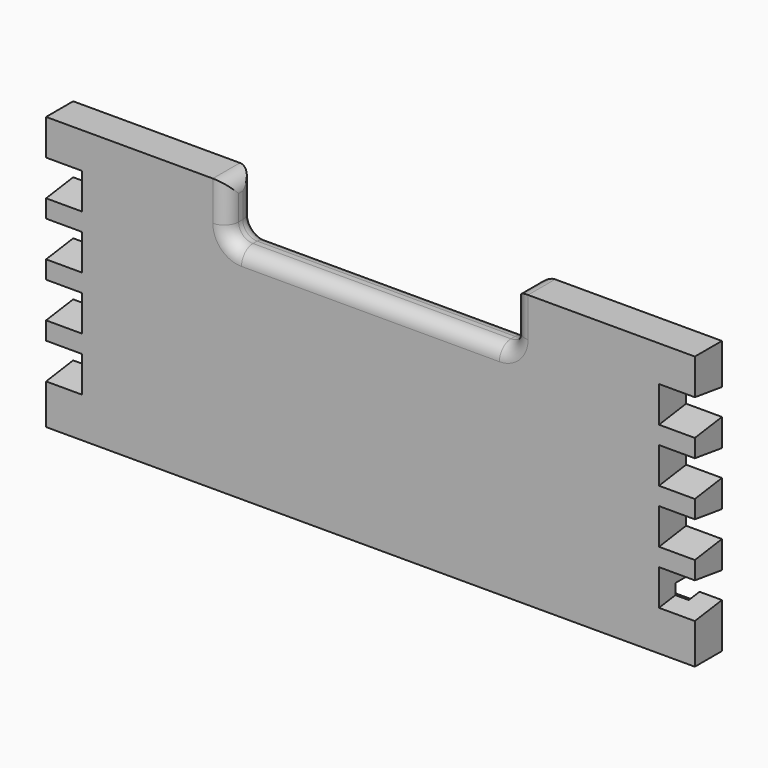
from build123d import *

# Parameters (mm, degrees)
F0_W     = 230
F0_H     = 96.8045385678
F1_DEPTH = 12
F2_W     = 101.6
F2_H     = 19.05
F3_DEPTH = 12
F4_R     = 5.08
F6_DEPTH = 12.7
F7_W     = 204.6
F7_H     = 6.35
F7_W_2   = 4.7625
F8_DEPTH = 4.7625


# Not quite as in the source:
# - a pattern or mirror of a feature is missing from the dataset's text; its kind, count and spacing are read off the source's solid


with BuildPart() as f1:
    # F0 (on Front) → F1 (new body)
    with BuildSketch(Plane.XZ):
        Rectangle(F0_W, F0_H)
    extrude(amount=-F1_DEPTH)

    # F2 (on face) → F3 (cut, through all)
    with BuildSketch(Plane.XZ):
        with Locations((0, 38.8772692839)):
            Rectangle(F2_W, F2_H)
    extrude(amount=-F3_DEPTH, mode=Mode.SUBTRACT)

    # F4
    f4_edges = [f1.edges().sort_by_distance(p)[0] for p in [
        (-50.8, 6, 48.402269),
        (-50.8, 6, 29.352269),
        (-50.8, 0, 38.877269),
        (-50.8, 12, 38.877269),
        (50.8, 6, 29.352269),
        (50.8, 6, 48.402269),
        (50.8, 0, 38.877269),
        (50.8, 12, 38.877269),
        (0, 0, 29.352269),
        (0, 12, 29.352269),
    ]]
    fillet(f4_edges, radius=F4_R)

    # F5 (on face) → F6 (cut)
    with BuildSketch(Plane.YZ.offset(115)):
        Polygon((12, 34.0157792675), (0, 35.7022692839), (0, 23.0022692839), (12, 24.6887593003), align=None)
        Polygon((12, 14.9657792675), (0, 16.6522692839), (0, 3.9522692839), (12, 5.6387593003), align=None)
        Polygon((12, -4.0842207325), (0, -2.3977307161), (0, -15.0977307161), (12, -13.4112406997), align=None)
        Polygon((12, -23.1342207325), (0, -21.4477307161), (0, -34.1477307161), (12, -32.4612406997), align=None)
    f6 = extrude(amount=-F6_DEPTH, mode=Mode.SUBTRACT)

    # F6_copies: F6 across plane
    add(f6.mirror(Plane(origin=(0, 0, 0), x_dir=(0, 0, -1), z_dir=(-1, 0, 0))), mode=Mode.SUBTRACT)

    # F7 (on face) → F8 (cut)
    with BuildSketch(Plane(origin=(0, 12, 0), x_dir=(-1, 0, 0), z_dir=(0, 1, 0))):
        with Locations((0, -32.5272692839)):
            Rectangle(F7_W, F7_H)
        with Locations((-104.68125, -32.5272692839)):
            Rectangle(F7_W_2, F7_H)
        with Locations((104.68125, -32.5272692839)):
            Rectangle(F7_W_2, F7_H)
    extrude(amount=-F8_DEPTH, mode=Mode.SUBTRACT)


solid = f1.part
